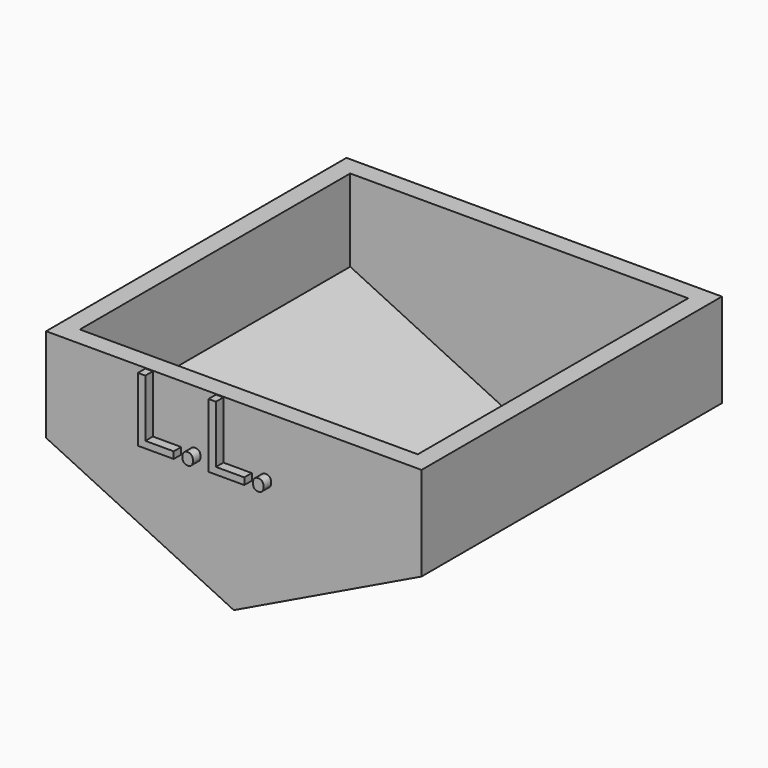
from build123d import *

# Parameters (mm, degrees)
F1_DEPTH     = 50.8
F2_T         = -2.54
F3_TEXT_SIZE = 12.1637514803
F4_DEPTH     = 1.27


# Not quite as in the source:
# - Text() gives the source's letters only with a copy of the font that has no kerning and outlines rounded to 1/6400 em; it was checked with that copy


with BuildPart() as f1:
    # F0 (on Front) → F1 (new body)
    with BuildSketch(Plane.XZ):
        Polygon((-13.2956014395, 8.7579010658), (-64.0956014395, 8.7579010658), (-64.0956014395, -3.9420989342), (-38.6956014395, -16.2064060569), (-13.2956014395, -3.9420989342), align=None)
    extrude(amount=F1_DEPTH)

    # F2
    f2_openings = [f1.faces().sort_by_distance(p)[0] for p in [
        (-38.695601, -25.4, 8.757901),
    ]]
    offset(amount=F2_T, openings=f2_openings)

    # F3 (on face) → F4 (join)
    with BuildSketch(Plane.XZ.offset(50.8)):
        with Locations((-51.8493242562, 0)):
            Text('L.L.', F3_TEXT_SIZE, font='Open Sans', text_align=(TextAlign.LEFT, TextAlign.BOTTOM))
    extrude(amount=F4_DEPTH)


solid = f1.part
